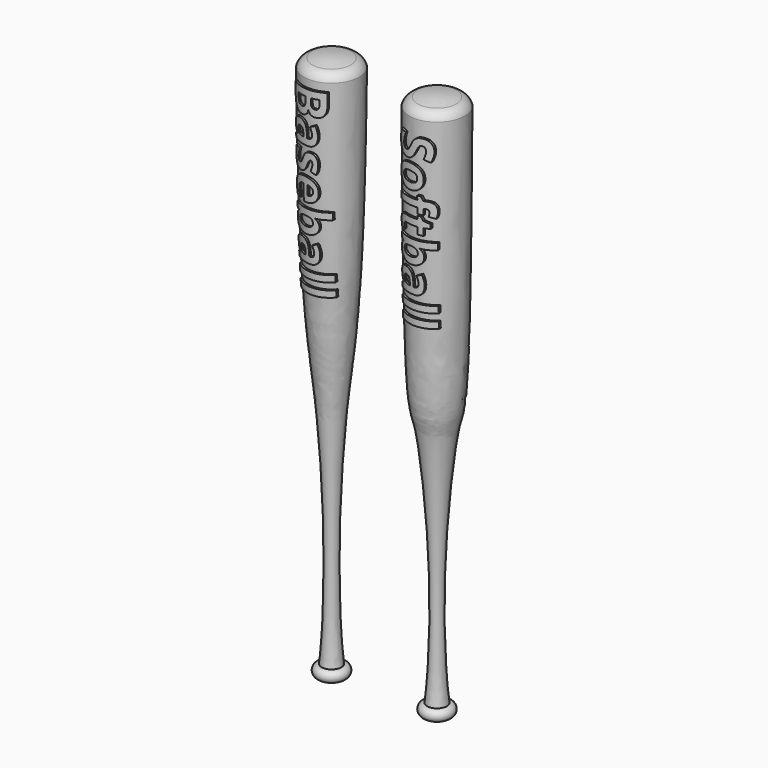
from build123d import *

# Parameters (mm, degrees)
F1_TEXT_SIZE = 4.2580572578
F3_DEPTH     = 2.8
F7_DEPTH     = 25


# Not quite as in the source:
# - Text() gives the source's letters only with a copy of the font that has no kerning and outlines rounded to 1/6400 em; it was checked with that copy


with BuildPart() as f2:
    # F0 (on Front) → F2 (revolve)
    with BuildSketch(Plane.XZ):
        with BuildLine():
            add(Edge.make_bspline(
                [(6.4795200313, 24.7643647223), (6.3241149799, -2.7930190555), (5.8057404319, 3.1596030486), (4.1800676024, -13.6339855295), (4.4855855033, -21.8251474676), (4.7947384599, -24.6693545281)],
                knots=[0, 0, 0, 0, 0.4365051354, 0.7160286605, 1, 1, 1, 1], degree=3))
            ThreePointArc((6.4795200313, 24.7643647223), (6.1768571097, 25.236842976), (5.6817147714, 25.5008024602))
            ThreePointArc((5.6817147714, 25.5008024602), (4.7852221458, 25.6808765497), (3.8728184598, 25.7412522023))
            Line((3.8728184598, 25.7412522023), (3.8728184598, 24.9358266592))
            Line((3.8728184598, 24.9358266592), (3.8728184598, -25.7189328344))
            Line((3.8728184598, -25.7189328344), (4.7947384599, -25.7189328344))
            ThreePointArc((4.7947384599, -25.7189328344), (5.3254262134, -25.1941436813), (4.7947384599, -24.6693545281))
        make_face()
    revolve(axis=Axis((3.8728184598, 0, -0.3915530876), (0, 0, -1)))

    # F1 (on Front) → F3 (intersect)
    with BuildSketch(Plane.XZ):
        with Locations(Location((2.3599714041, 23.6163324397), (0, 0, -90))):
            Text('Softball', F1_TEXT_SIZE, font='Open Sans', font_style=FontStyle.BOLD, text_align=(TextAlign.LEFT, TextAlign.BOTTOM))
        with Locations(Location((-7.606210705, 24.409395604), (0, 0, -90))):
            Text('Baseball', F1_TEXT_SIZE, font='Open Sans', font_style=FontStyle.BOLD, text_align=(TextAlign.LEFT, TextAlign.BOTTOM))
    extrude(amount=F3_DEPTH, mode=Mode.INTERSECT)


with BuildPart() as f2_1:
    # F4: moved
    add(f2.part.moved(Location((0, -0.2, 0))))

    # F0 (on Front) → F5 (revolve)
    with BuildSketch(Plane.XZ):
        with BuildLine():
            add(Edge.make_bspline(
                [(6.4795200313, 24.7643647223), (6.3241149799, -2.7930190555), (5.8057404319, 3.1596030486), (4.1800676024, -13.6339855295), (4.4855855033, -21.8251474676), (4.7947384599, -24.6693545281)],
                knots=[0, 0, 0, 0, 0.4365051354, 0.7160286605, 1, 1, 1, 1], degree=3))
            ThreePointArc((6.4795200313, 24.7643647223), (6.1768571097, 25.236842976), (5.6817147714, 25.5008024602))
            ThreePointArc((5.6817147714, 25.5008024602), (4.7852221458, 25.6808765497), (3.8728184598, 25.7412522023))
            Line((3.8728184598, 25.7412522023), (3.8728184598, 24.9358266592))
            Line((3.8728184598, 24.9358266592), (3.8728184598, -25.7189328344))
            Line((3.8728184598, -25.7189328344), (4.7947384599, -25.7189328344))
            ThreePointArc((4.7947384599, -25.7189328344), (5.3254262134, -25.1941436813), (4.7947384599, -24.6693545281))
        make_face()
    revolve(axis=Axis((3.8728184598, 0, -0.3915530876), (0, 0, -1)))


with BuildPart() as f6:
    # F0 (on Front) → F6 (revolve)
    with BuildSketch(Plane.XZ):
        with BuildLine():
            add(Edge.make_bspline(
                [(-3.4411179651, 24.7643647223), (-3.6326580149, 5.1531886189), (-4.7209022947, 0.3143089908), (-5.5918952083, -13.0724183033), (-5.4295679547, -21.8194323144), (-5.1197937857, -24.6693545281)],
                knots=[0, 0, 0, 0, 0.4406263754, 0.7154580481, 1, 1, 1, 1], degree=3))
            ThreePointArc((-3.4411179651, 24.7643647223), (-3.7437808867, 25.236842976), (-4.238923225, 25.5008024602))
            ThreePointArc((-4.238923225, 25.5008024602), (-5.1354158506, 25.6808765497), (-6.0478195366, 25.7412522023))
            Line((-6.0478195366, 25.7412522023), (-6.0478195366, -25.7189328344))
            Line((-6.0478195366, -25.7189328344), (-5.1197937857, -25.7189328344))
            ThreePointArc((-5.1197937857, -25.7189328344), (-4.5891060322, -25.1941436813), (-5.1197937857, -24.6693545281))
        make_face()
    revolve(axis=Axis((-6.0478195366, 0, 0.0111596839), (0, 0, -1)))

    # F1 (on Front) → F7 (intersect)
    with BuildSketch(Plane.XZ):
        with Locations(Location((-7.606210705, 24.409395604), (0, 0, -90))):
            Text('Baseball', F1_TEXT_SIZE, font='Open Sans', font_style=FontStyle.BOLD, text_align=(TextAlign.LEFT, TextAlign.BOTTOM))
    extrude(amount=F7_DEPTH, mode=Mode.INTERSECT)


with BuildPart() as f6_1:
    # F8: moved
    add(f6.part.moved(Location((0, -0.2, 0))))

    # F0 (on Front) → F9 (revolve)
    with BuildSketch(Plane.XZ):
        with BuildLine():
            add(Edge.make_bspline(
                [(-3.4411179651, 24.7643647223), (-3.6326580149, 5.1531886189), (-4.7209022947, 0.3143089908), (-5.5918952083, -13.0724183033), (-5.4295679547, -21.8194323144), (-5.1197937857, -24.6693545281)],
                knots=[0, 0, 0, 0, 0.4406263754, 0.7154580481, 1, 1, 1, 1], degree=3))
            ThreePointArc((-3.4411179651, 24.7643647223), (-3.7437808867, 25.236842976), (-4.238923225, 25.5008024602))
            ThreePointArc((-4.238923225, 25.5008024602), (-5.1354158506, 25.6808765497), (-6.0478195366, 25.7412522023))
            Line((-6.0478195366, 25.7412522023), (-6.0478195366, -25.7189328344))
            Line((-6.0478195366, -25.7189328344), (-5.1197937857, -25.7189328344))
            ThreePointArc((-5.1197937857, -25.7189328344), (-4.5891060322, -25.1941436813), (-5.1197937857, -24.6693545281))
        make_face()
    revolve(axis=Axis((-6.0478195366, 0, 0.0111596839), (0, 0, -1)))


solid = Compound([f2_1.part, f6_1.part])
